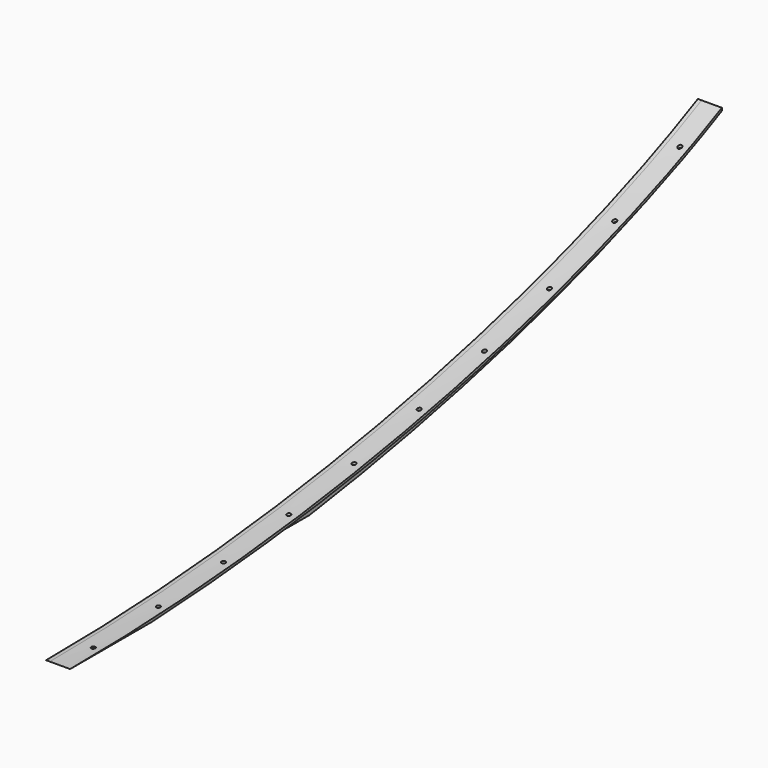
from build123d import *

# Parameters (mm, degrees)
F1_DEPTH      = 25
F1_DEPTH_BACK = 4.5
F2_DEPTH      = 4.5
F3_DEPTH      = 1.5
F4_R          = 2.5
F5_DEPTH      = 150
F6_R          = 4.1800646045
F7_DEPTH      = 12.5


# Not quite as in the source:
# - the dataset's text gives a spline's control points without its knots; the knots are read off the source's solid


with BuildPart() as f1:
    # F0 (on Right) → F1 (new body, two sides)
    with BuildSketch(Plane.YZ) as f1_sk:
        with BuildLine():
            add(Edge.make_bspline(
                [(-542.9529296271, -39.9508323044), (-188.0693441655, -39.9508323044), (204.5968802247, 34.2876766354), (457.0470703729, 160.0491676956)],
                knots=[0, 0, 0, 0, 1019.8039027186, 1019.8039027186, 1019.8039027186, 1019.8039027186], degree=3))
            Line((-542.9529296271, -39.9508323044), (-417.3127151335, -39.9508323044))
            add(Edge.make_bspline(
                [(-417.3127151335, -39.9508323044), (-369.1001563129, -37.6799090107), (-229.605831227, -27.4883990926), (-0.7659143619, 6.0089411279), (250.4802761754, 69.14721948), (394.0857076642, 125.4398419701), (457.047070373, 156.6986558412)],
                knots=[0.116693999, 0.116693999, 0.116693999, 0.116693999, 0.25, 0.5, 0.75, 0.9982402372, 0.9982402372, 0.9982402372, 0.9982402372], degree=3))
            Line((457.0470703729, 156.6986558412), (457.0470703729, 160.0491676956))
        make_face()
    extrude(amount=F1_DEPTH)
    extrude(f1_sk.sketch, amount=-F1_DEPTH_BACK)

    # F0 (on Right) → F2 (join, symmetric)
    with BuildSketch(Plane.YZ):
        with BuildLine():
            add(Edge.make_bspline(
                [(-417.3127151335, -39.9508323044), (-369.1001563129, -37.6799090107), (-229.605831227, -27.4883990926), (-0.7659143619, 6.0089411279), (250.4802761754, 69.14721948), (394.0857076642, 125.4398419701), (457.047070373, 156.6986558412)],
                knots=[0.116693999, 0.116693999, 0.116693999, 0.116693999, 0.25, 0.5, 0.75, 0.9982402372, 0.9982402372, 0.9982402372, 0.9982402372], degree=3))
            Line((-417.3127151335, -39.9508323044), (-149.937543661, -39.9508323044))
            add(Edge.make_bspline(
                [(-149.937543661, -39.9508323044), (-98.996798705, -32.7943859429), (-3.7016307054, -16.778446645), (131.246444394, 13.3933570474), (254.1058325956, 48.1234806847), (363.3774188375, 86.6936370443), (428.3490574687, 114.995507991), (457.0470703729, 128.861665731)],
                knots=[0.3594995159, 0.3594995159, 0.3594995159, 0.3594995159, 0.5, 0.625, 0.75, 0.875, 0.9840561675, 0.9840561675, 0.9840561675, 0.9840561675], degree=3))
            Line((457.0470703729, 128.861665731), (457.0470703729, 156.6986558412))
        make_face()
    extrude(amount=F2_DEPTH, both=True)

    # F0 (on Right) → F3 (cut, symmetric)
    with BuildSketch(Plane.YZ):
        with BuildLine():
            add(Edge.make_bspline(
                [(-417.3127151335, -39.9508323044), (-369.1001563129, -37.6799090107), (-229.605831227, -27.4883990926), (-0.7659143619, 6.0089411279), (250.4802761754, 69.14721948), (394.0857076642, 125.4398419701), (457.047070373, 156.6986558412)],
                knots=[0.116693999, 0.116693999, 0.116693999, 0.116693999, 0.25, 0.5, 0.75, 0.9982402372, 0.9982402372, 0.9982402372, 0.9982402372], degree=3))
            Line((-417.3127151335, -39.9508323044), (-149.937543661, -39.9508323044))
            add(Edge.make_bspline(
                [(-149.937543661, -39.9508323044), (-98.996798705, -32.7943859429), (-3.7016307054, -16.778446645), (131.246444394, 13.3933570474), (254.1058325956, 48.1234806847), (363.3774188375, 86.6936370443), (428.3490574687, 114.995507991), (457.0470703729, 128.861665731)],
                knots=[0.3594995159, 0.3594995159, 0.3594995159, 0.3594995159, 0.5, 0.625, 0.75, 0.875, 0.9840561675, 0.9840561675, 0.9840561675, 0.9840561675], degree=3))
            Line((457.0470703729, 128.861665731), (457.0470703729, 156.6986558412))
        make_face()
    extrude(amount=F3_DEPTH, both=True, mode=Mode.SUBTRACT)

    # F4 (on Top) → F5 (cut, symmetric)
    with BuildSketch(Plane.XY):
        with Locations((15, -494.9529296271)):
            Circle(F4_R)
        with Locations((15, -394.9529296271)):
            Circle(F4_R)
        with Locations((15, -294.9529296271)):
            Circle(F4_R)
        with Locations((15, -194.9529296271)):
            Circle(F4_R)
        with Locations((15, -94.9529296271)):
            Circle(F4_R)
        with Locations((15, 5.0470703729)):
            Circle(F4_R)
        with Locations((15, 105.0470703729)):
            Circle(F4_R)
        with Locations((15, 205.0470703729)):
            Circle(F4_R)
        with Locations((15, 305.0470703729)):
            Circle(F4_R)
        with Locations((15, 405.0470703729)):
            Circle(F4_R)
        with Locations((-15, -494.9529296271)):
            Circle(F4_R)
        with Locations((-15, -394.9529296271)):
            Circle(F4_R)
        with Locations((-15, -294.9529296271)):
            Circle(F4_R)
        with Locations((-15, -194.9529296271)):
            Circle(F4_R)
        with Locations((-15, -94.9529296271)):
            Circle(F4_R)
        with Locations((-15, 5.0470703729)):
            Circle(F4_R)
        with Locations((-15, 105.0470703729)):
            Circle(F4_R)
        with Locations((-15, 205.0470703729)):
            Circle(F4_R)
        with Locations((-15, 305.0470703729)):
            Circle(F4_R)
        with Locations((-15, 405.0470703729)):
            Circle(F4_R)
    extrude(amount=F5_DEPTH, both=True, mode=Mode.SUBTRACT)

    # F6 (on Right) → F7 (cut, symmetric)
    with BuildSketch(Plane.YZ):
        with Locations((442.0470703729, 131.861665731)):
            Circle(F6_R)
        with Locations((358.44841201, 95.9379511725)):
            Circle(F6_R)
        with Locations((273.163023997, 64.2259417875)):
            Circle(F6_R)
        with Locations((186.4029392463, 36.8044786279)):
            Circle(F6_R)
        with Locations((98.3838569987, 13.7417357717)):
            Circle(F6_R)
        with Locations((9.3246065611, -4.9049491686)):
            Circle(F6_R)
        with Locations((-80.5533967375, -19.0892175961)):
            Circle(F6_R)
        with Locations((-171.0267020195, -28.7758051847)):
            Circle(F6_R)
    extrude(amount=F7_DEPTH, both=True, mode=Mode.SUBTRACT)


solid = f1.part
